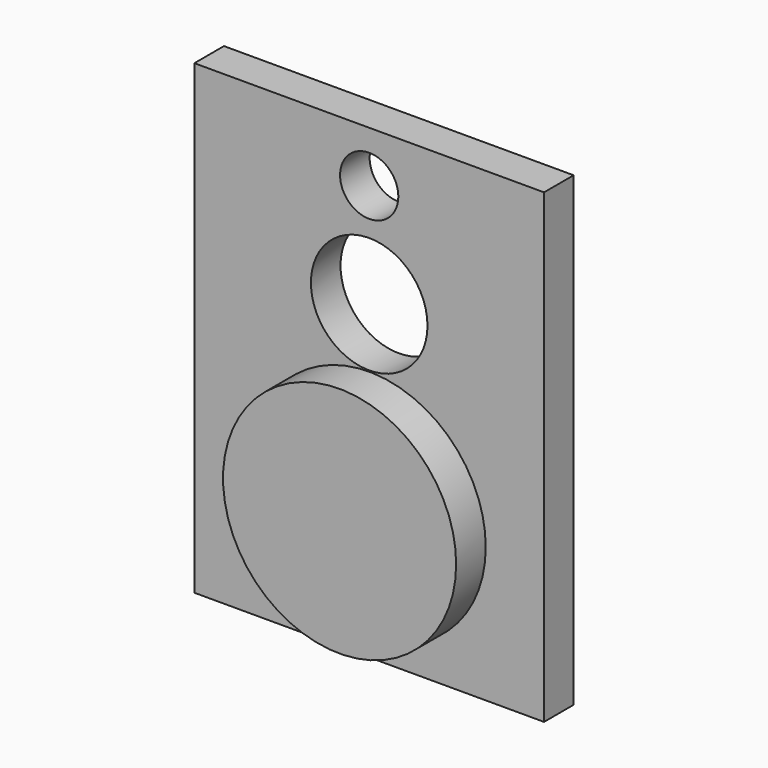
from build123d import *

# Parameters (mm, degrees)
F0_W     = 60
F0_H     = 80
F0_R     = 20
F0_R_2   = 10
F0_R_3   = 5
F1_DEPTH = 6.35
F2_DEPTH = 12.7


# Not quite as in the source:
# - a feature names something its author has since deleted; it is built from what else it names


with BuildPart() as f1:
    # F0 (on Front) → F1 (new body)
    with BuildSketch(Plane.XZ):
        Rectangle(F0_W, F0_H)
        with Locations((0, -16.8533538189)):
            Circle(F0_R, mode=Mode.SUBTRACT)
        with Locations((0, 13.3463527084)):
            Circle(F0_R_2, mode=Mode.SUBTRACT)
        with Locations((0, 31.2290439901)):
            Circle(F0_R_3, mode=Mode.SUBTRACT)
    extrude(amount=F1_DEPTH)

    # F0 (on Front) → F2 (join)
    with BuildSketch(Plane.XZ):
        with Locations((0, -16.8533538189)):
            Circle(F0_R)
    extrude(amount=F2_DEPTH)


solid = f1.part
